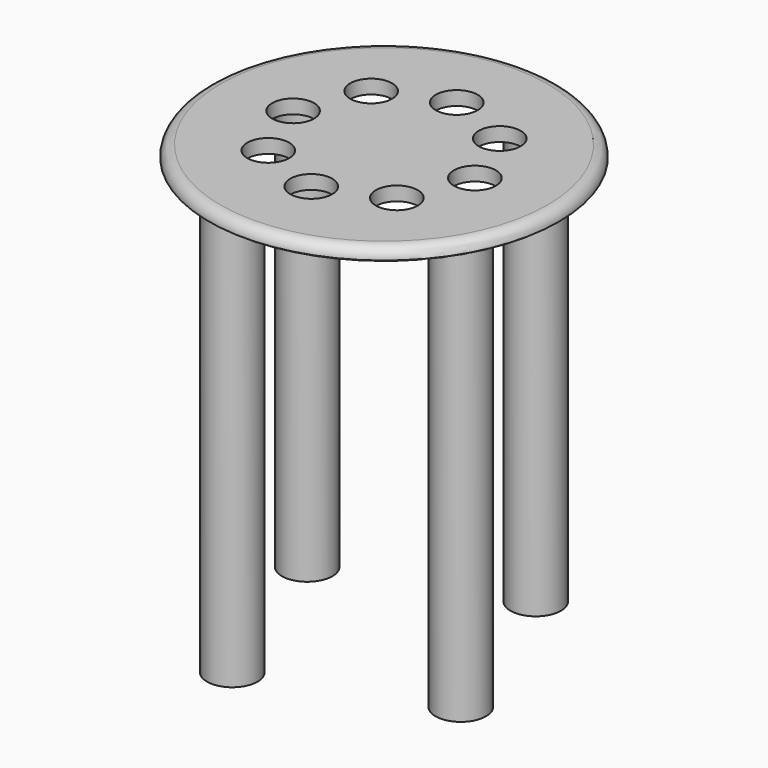
from build123d import *

# Parameters (mm, degrees)
F0_R     = 125
F2_DEPTH = 10
F1_R     = 15
F3_DEPTH = 39
F4_DEPTH = 107
F5_R     = 8
F7_R     = 18.065377162
F8_DEPTH = 300


# Not quite as in the source:
# - a fillet or chamfer that OpenCascade refuses, or shapes differently, is made with other operations: its cross-section is extruded or revolved along the edge and cut away or added


with BuildPart() as f2:
    # F0 (on Top) → F2 (new body)
    with BuildSketch(Plane.XY):
        Circle(F0_R)
    extrude(amount=F2_DEPTH)

    # F1 (on face) → F3 (join)
    with BuildSketch(Plane.XY):
        with Locations((-45.9619407771, -45.9619407771)):
            Circle(F1_R)
        with Locations((-65, 0)):
            Circle(F1_R)
        with Locations((0, 65)):
            Circle(F1_R)
        with Locations((0, -65)):
            Circle(F1_R)
        with Locations((45.9619407771, -45.9619407771)):
            Circle(F1_R)
        with Locations((65, 0)):
            Circle(F1_R)
        with Locations((45.9619407771, 45.9619407771)):
            Circle(F1_R)
        with Locations((-45.9619407771, 45.9619407771)):
            Circle(F1_R)
    extrude(amount=F3_DEPTH)

    # F4 (cut): faces of the model
    f4_faces = [f2.faces().sort_by_distance(p)[0] for p in [
        (-45.9619407771, -45.9619407771, 39),
        (0, -65, 39),
        (45.9619407771, -45.9619407771, 39),
        (65, 0, 39),
        (45.9619407771, 45.9619407771, 39),
        (0, 65, 39),
        (-45.9619407771, 45.9619407771, 39),
        (-65, 0, 39),
    ]]
    extrude(f4_faces, amount=-F4_DEPTH, mode=Mode.SUBTRACT)

    # F5
    f5_edges = [f2.edges().sort_by_distance(p)[0] for p in [
        (-125, 0, 10),
    ]]
    fillet(f5_edges, radius=F5_R)

    # F6: fillet of radius 8 on 1 edges, made by hand

    # F6_s1 → F6_t2 (revolve, cut)
    with BuildSketch(Plane.XZ):
        with BuildLine():
            ThreePointArc((125, 2), (122.5369245026, 0.5166852265), (119.7084973779, 0))
            Line((119.7084973779, 0), (125, 0))
            Line((125, 0), (125, 2))
        make_face()
    revolve(axis=Axis((0, 0, 0), (0, 0, 1)), mode=Mode.SUBTRACT)

    # F7 (on face) → F8 (join)
    with BuildSketch(Plane(origin=(0, 0, 0), x_dir=(1, 0, 0), z_dir=(0, 0, -1))):
        with Locations((39.3640957773, -86.4013507962)):
            Circle(F7_R)
        with Locations((-86.4013507962, -39.3640957773)):
            Circle(F7_R)
        with Locations((-39.3640957773, 86.4013507962)):
            Circle(F7_R)
        with Locations((86.4013507962, 39.3640957773)):
            Circle(F7_R)
    extrude(amount=F8_DEPTH)


solid = f2.part
